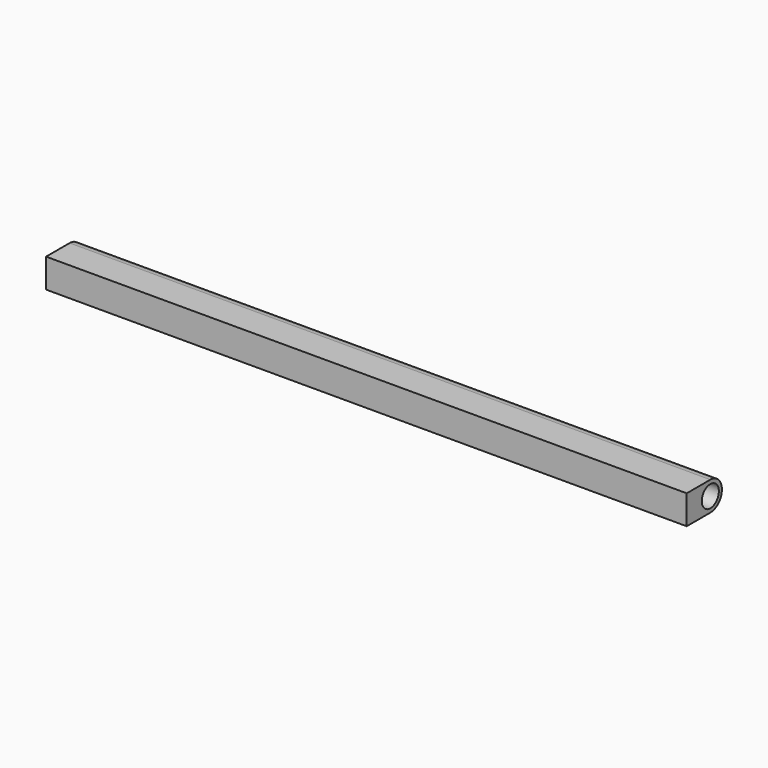
from build123d import *

# Parameters (mm, degrees)
F0_W     = 150
F0_H     = 10.3
F1_DEPTH = 6.8
F2_R     = 3.39999
F3_R     = 2.5
F4_DEPTH = 150.001


# Not quite as in the source:
# - a fillet or chamfer is up to 0.001 mm smaller than in the source, because OpenCascade refuses the exact size


with BuildPart() as f1:
    # F0 (on Top) → F1 (new body)
    with BuildSketch(Plane.XY):
        with Locations((47.3209783435, -1.7712331437)):
            Rectangle(F0_W, F0_H)
    extrude(amount=F1_DEPTH)

    # F2 (radius 3.4 in the source; OpenCascade refuses exactly that, so slightly less here)
    f2_edges = [f1.edges().sort_by_distance(p)[0] for p in [
        (47.320978, 3.378767, 6.8),
        (47.320978, 3.378767, 0),
    ]]
    fillet(f2_edges, radius=F2_R)

    # F3 (on face) → F4 (cut, through all)
    with BuildSketch(Plane(origin=(-27.6790216565, 0, 0), x_dir=(0, -1, 0), z_dir=(-1, 0, 0))):
        with Locations((0.0212331437, 3.4)):
            Circle(F3_R)
    extrude(amount=-F4_DEPTH, mode=Mode.SUBTRACT)


solid = f1.part
